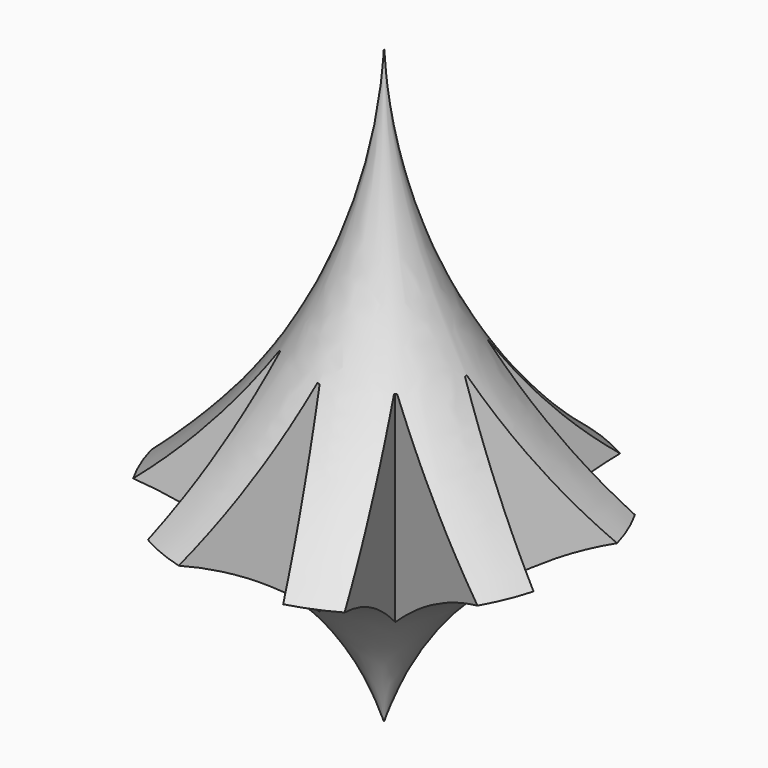
from build123d import *

# Parameters (mm, degrees)
F3_DEPTH        = 33.4
F3_COPIES_COUNT = 8


# Not quite as in the source:
# - a pattern or mirror of a feature is missing from the dataset's text; its kind, count and spacing are read off the source's solid


with BuildPart() as f1:
    # F0 (on Front) → F1 (revolve)
    with BuildSketch(Plane.XZ):
        with BuildLine():
            ThreePointArc((0, 0), (7.4950834983, 12.5049165017), (20, 20))
            ThreePointArc((20, 20), (5.7509146035, 37.8754573017), (0, 60))
            Line((0, 60), (0, 0))
        make_face()
    revolve(axis=Axis((0, 0, 15.3403095348), (0, 0, 1)))

    # F2 (on Top) → F3 (cut)
    with BuildSketch(Plane.XY):
        with BuildLine():
            Line((0, 8), (5.2665405035, 19.2941325569))
            ThreePointArc((5.2665405035, 19.2941325569), (0, 20), (-5.2665405035, 19.2941325569))
            Line((-5.2665405035, 19.2941325569), (0, 8))
        make_face()
    f3 = extrude(amount=F3_DEPTH, mode=Mode.SUBTRACT)

    # F3_copies: F3 ×8 about axis
    f3_copies_axis = Axis((0, 0, 0), (0, 0, 1))
    for i in range(1, F3_COPIES_COUNT):
        add(f3.rotate(f3_copies_axis, i * 360 / F3_COPIES_COUNT), mode=Mode.SUBTRACT)


solid = f1.part
